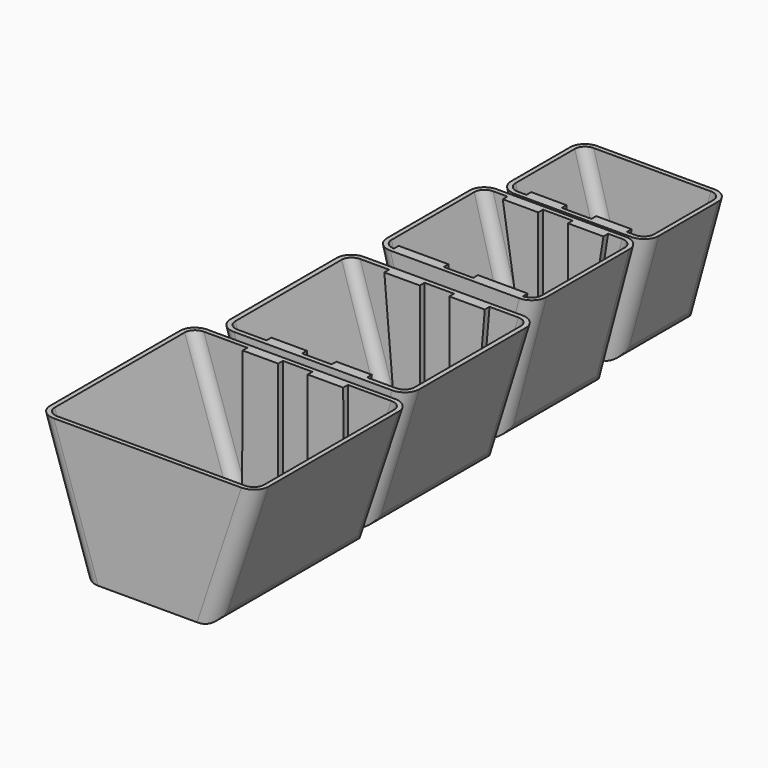
from build123d import *

# Parameters (mm, degrees)
F1_DEPTH  = 65
F2_R      = 5
F5_DEPTH  = 55
F6_R      = 5
F9_DEPTH  = 45
F10_R     = 5
F13_DEPTH = 35
F14_R     = 5
F15_T     = -1.6
F16_T     = -1.5
F17_T     = -1.5
F18_T     = -1.5
F20_DEPTH = 2
F22_DEPTH = 2
F24_DEPTH = 2
F26_DEPTH = 2
F28_DEPTH = 2
F30_DEPTH = 2


# Not quite as in the source:
# - a feature names something its author has since deleted; it is built from what else it names


with BuildPart() as f1:
    # F0 (on Front) → F1 (new body)
    with BuildSketch(Plane.XZ):
        Polygon((37, 23.9011184353), (0, 23.9011184353), (-37, 23.9011184353), (-22, -21.0988815647), (0, -21.0988815647), (22, -21.0988815647), align=None)
    extrude(amount=F1_DEPTH)

    # F2
    f2_edges = [f1.edges().sort_by_distance(p)[0] for p in [
        (-22, -32.5, -21.098882),
        (22, -32.5, -21.098882),
        (-29.5, -65, 1.401118),
        (29.5, -65, 1.401118),
        (29.5, 0, 1.401118),
        (-29.5, 0, 1.401118),
    ]]
    fillet(f2_edges, radius=F2_R)

    # F17
    f17_openings = [f1.faces().sort_by_distance(p)[0] for p in [
        (0, -32.5, 23.901118),
    ]]
    offset(amount=F17_T, openings=f17_openings)

    # F29 (on face) → F30 (join)
    with BuildSketch(Plane.XZ.offset(1.5)):
        Polygon((-5, -19.5988815647), (-5, 23.9011184353), (-17, 23.9011184353), (-17.2295372331, -19.5988815647), align=None)
        Polygon((17, 23.9011184353), (5, 23.9011184353), (5, -19.5988815647), (17.2295372331, -19.5988815647), align=None)
    extrude(amount=F30_DEPTH)


with BuildPart() as f5:
    # F4 (on offset) → F5 (new body)
    with BuildSketch(Plane.XZ.offset(-60)):
        Polygon((32, 22.8169034502), (0, 22.8169034502), (-32, 22.8169034502), (-18, -22.1830965498), (0, -22.1830965498), (18, -22.1830965498), align=None)
    extrude(amount=F5_DEPTH)

    # F6
    f6_edges = [f5.edges().sort_by_distance(p)[0] for p in [
        (25, 60, 0.316903),
        (-25, 60, 0.316903),
        (18, 32.5, -22.183097),
        (-18, 32.5, -22.183097),
        (-25, 5, 0.316903),
        (25, 5, 0.316903),
    ]]
    fillet(f6_edges, radius=F6_R)

    # F15
    f15_openings = [f5.faces().sort_by_distance(p)[0] for p in [
        (0, 32.5, 22.816903),
    ]]
    offset(amount=F15_T, openings=f15_openings)

    # F25 (on face) → F26 (join)
    with BuildSketch(Plane.XZ.offset(-58.4)):
        Polygon((-5, -20.5830965498), (-5, 22.8169034502), (-17, 22.8169034502), (-13.2613903698, -20.5830965498), align=None)
        Polygon((17, 22.8169034502), (5, 22.8169034502), (5, -20.5830965498), (13.2613903698, -20.5830965498), align=None)
    extrude(amount=F26_DEPTH)

    # F27 (on face) → F28 (join)
    with BuildSketch(Plane(origin=(0, 6.6, 0), x_dir=(-1, 0, 0), z_dir=(0, 1, 0))):
        Polygon((5, 22.8169034502), (5, -20.5830965498), (13.2613903698, -20.5830965498), (17, 22.8169034502), align=None)
        Polygon((-13.2613903698, -20.5830965498), (-5, -20.5830965498), (-5, 22.8169034502), (-17, 22.8169034502), align=None)
    extrude(amount=F28_DEPTH)


with BuildPart() as f9:
    # F8 (on offset) → F9 (new body)
    with BuildSketch(Plane.XZ.offset(-110)):
        Polygon((27, 24.2408766891), (0, 24.2408766891), (-27, 24.2408766891), (-15, -20.7591233109), (0, -20.7591233109), (15, -20.7591233109), align=None)
    extrude(amount=F9_DEPTH)

    # F10
    f10_edges = [f9.edges().sort_by_distance(p)[0] for p in [
        (21, 110, 1.740877),
        (-21, 110, 1.740877),
        (15, 87.5, -20.759123),
        (-15, 87.5, -20.759123),
        (21, 65, 1.740877),
        (-21, 65, 1.740877),
    ]]
    fillet(f10_edges, radius=F10_R)

    # F18
    f18_openings = [f9.faces().sort_by_distance(p)[0] for p in [
        (0, 87.5, 24.240877),
    ]]
    offset(amount=F18_T, openings=f18_openings)

    # F19 (on face) → F20 (join)
    with BuildSketch(Plane.XZ.offset(-108.5)):
        Polygon((-10.2252751012, -19.2591233109), (-5, -19.2591233109), (-5, 24.2408766891), (-17, 24.2408766891), align=None)
        Polygon((5.0505502025, 24.2408766891), (5.0505502025, -19.2591233109), (10.2252751012, -19.2591233109), (10.346798193, -18.8034117168), (17.0505502025, 24.2408766891), align=None)
    extrude(amount=F20_DEPTH)

    # F21 (on face) → F22 (join)
    with BuildSketch(Plane(origin=(0, 66.5, 0), x_dir=(-1, 0, 0), z_dir=(0, 1, 0))):
        Polygon((-10.2252751012, -19.2591233109), (-5, -19.2591233109), (-5, 24.2408766891), (-21.8252751012, 24.2408766891), align=None)
        Polygon((5, -19.2591233109), (10.2252751012, -19.2591233109), (21.8252751012, 24.2408766891), (5, 24.2408766891), align=None)
    extrude(amount=F22_DEPTH)


with BuildPart() as f13:
    # F12 (on offset) → F13 (new body)
    with BuildSketch(Plane.XZ.offset(-150)):
        Polygon((25, 21.4980914434), (0, 21.4980914434), (-25, 21.4980914434), (-14, -18.5019085566), (0, -18.5019085566), (14, -18.5019085566), align=None)
    extrude(amount=F13_DEPTH)

    # F14
    f14_edges = [f13.edges().sort_by_distance(p)[0] for p in [
        (19.5, 150, 1.498091),
        (-19.5, 150, 1.498091),
        (14, 132.5, -18.501909),
        (-14, 132.5, -18.501909),
        (19.5, 115, 1.498091),
        (-19.5, 115, 1.498091),
    ]]
    fillet(f14_edges, radius=F14_R)

    # F16
    f16_openings = [f13.faces().sort_by_distance(p)[0] for p in [
        (0, 132.5, 21.498091),
    ]]
    offset(amount=F16_T, openings=f16_openings)

    # F23 (on face) → F24 (join)
    with BuildSketch(Plane(origin=(0, 116.5, 0), x_dir=(-1, 0, 0), z_dir=(0, 1, 0))):
        Polygon((-10, -17.0019085566), (-5, -17.0019085566), (-5, 21.4980914434), (-17, 21.4980914434), align=None)
        Polygon((5, 21.4980914434), (5, -17.0019085566), (10, -17.0019085566), (17, 21.4980914434), align=None)
        Polygon((5, 21.4980914434), (5, -17.0019085566), (9.2268828718, -17.0019085566), (11.5085212257, -8.7050418152), (17, 21.4980914434), align=None)
    extrude(amount=F24_DEPTH)


solid = Compound([f1.part, f5.part, f9.part, f13.part])
